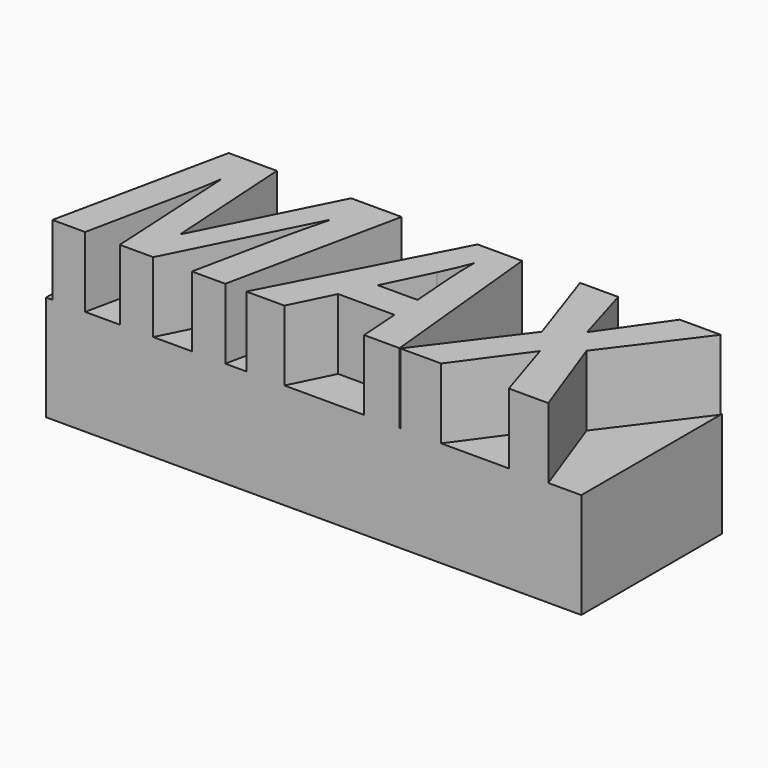
from build123d import *

# Parameters (mm, degrees)
F0_TEXT_SIZE = 21.1666666667
F1_DEPTH     = 9.144
F2_DEPTH     = 15.24


# Not quite as in the source:
# - Text() gives the source's letters only with a copy of the font that has no kerning and outlines rounded to 1/6400 em; it was checked with that copy


with BuildPart() as f1:
    # F0 (on Top) → F1 (new body)
    with BuildSketch(Plane.XY):
        Polygon((-23.19734375, 7.62), (-23.19734375, -7.62), (-22.6483333333, -7.62), (-19.456796875, 7.491015625), (-15.2796875, 7.491015625), (-14.5785416667, -3.8066927083), (-14.535546875, -3.8066927083), (-8.840390625, 7.491015625), (-4.4681510417, 7.491015625), (-7.6629947917, -7.62), (-5.843984375, -7.62), (2.0703645833, 7.5538541667), (5.9266666667, 7.5538541667), (7.4447135417, -7.62), (7.5075520833, -7.62), (13.4606770833, 0.2778125), (11.003359375, 7.491015625), (14.3106510417, 7.491015625), (15.8915364583, 2.1365104167), (19.6420052083, 7.491015625), (23.19734375, 7.491015625), (23.19734375, 7.62), align=None)
        with BuildLine():
            add(Edge.make_bspline(
                [(-17.8742578125, 1.7032552083), (-18.1537239583, 0.2248958333), (-19.8073697917, -7.62)],
                knots=[0, 0, 0, 1, 1, 1], degree=2))
            Line((-19.8073697917, -7.62), (-16.8109635417, -7.62))
            Line((-16.8109635417, -7.62), (-17.4393489583, 4.0911197917))
            Line((-17.4393489583, 4.0911197917), (-17.48234375, 4.0911197917))
            add(Edge.make_bspline(
                [(-17.48234375, 4.0911197917), (-17.5947916667, 3.1816145833), (-17.8742578125, 1.7032552083)],
                knots=[0, 0, 0, 1, 1, 1], degree=2))
        make_face()
        Polygon((23.19734375, -7.62), (23.19734375, 7.491015625), (17.5650260417, -0.0033072917), (20.3365364583, -7.62), align=None)
        with BuildLine():
            Line((-8.0234895833, 4.0911197917), (-13.9071614583, -7.62))
            Line((-13.9071614583, -7.62), (-10.556875, -7.62))
            Line((-10.556875, -7.62), (-9.058671875, -0.466328125))
            add(Edge.make_bspline(
                [(-9.058671875, -0.466328125), (-8.5096614583, 2.08359375), (-7.9738802083, 4.0911197917)],
                knots=[0, 0, 0, 1, 1, 1], degree=2))
            Line((-7.9738802083, 4.0911197917), (-8.0234895833, 4.0911197917))
        make_face()
        Polygon((11.043046875, -7.62), (16.9134895833, -7.62), (15.1374739583, -2.0075260417), align=None)
        with Locations((-23.19734375, -7.62)):
            Text('MAX', F0_TEXT_SIZE, font='Open Sans', font_style=FontStyle.BOLDITALIC, text_align=(TextAlign.LEFT, TextAlign.BOTTOM))
        Polygon((-0.7606770833, -4.0216666667), (-2.5366927083, -7.62), (4.375546875, -7.62), (4.1275, -4.0216666667), align=None)
        with BuildLine():
            Line((0.5324739583, -1.3361458333), (3.9720572917, -1.3361458333))
            Line((3.9720572917, -1.3361458333), (3.7041666667, 2.28203125))
            add(Edge.make_bspline(
                [(3.7041666667, 2.28203125), (3.601640625, 3.6347135417), (3.601640625, 4.8947916667)],
                knots=[0, 0, 0, 1, 1, 1], degree=2))
            Line((3.601640625, 4.8947916667), (3.601640625, 5.268515625))
            add(Edge.make_bspline(
                [(3.601640625, 5.268515625), (3.145234375, 4.02828125), (2.4738541667, 2.6425260417)],
                knots=[0, 0, 0, 1, 1, 1], degree=2))
            Line((2.4738541667, 2.6425260417), (0.5324739583, -1.3361458333))
        make_face()
    extrude(amount=F1_DEPTH)

    # F0 (on Top) → F2 (join)
    with BuildSketch(Plane.XY):
        with Locations((-23.19734375, -7.62)):
            Text('MAX', F0_TEXT_SIZE, font='Open Sans', font_style=FontStyle.BOLDITALIC, text_align=(TextAlign.LEFT, TextAlign.BOTTOM))
    extrude(amount=F2_DEPTH)


solid = f1.part
